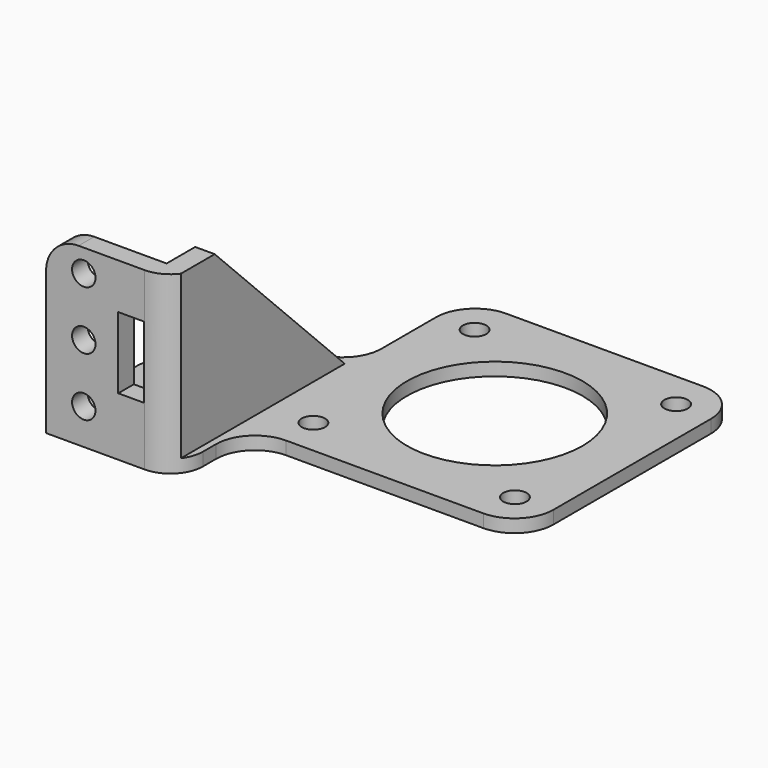
from build123d import *

# Parameters (mm, degrees)
F0_R         = 1.8
F0_R_2       = 13.5
F0_W         = 20.1372796029
F0_H         = 13.5
F1_DEPTH     = 2
F2_W         = 3
F2_H         = 33.5
F3_DEPTH     = 27
F4_W         = 16.1372796029
F4_H         = 3
F5_DEPTH     = 25
F6_R         = 1.8
F6_W         = 4
F6_H         = 11
F7_DEPTH     = 25
F8_SIZE      = 25
F9_SIZE      = 14
F10_R        = 5
F11_T1_DEPTH = 2
F11_T3_DEPTH = 32


# Not quite as in the source:
# - a fillet or chamfer that OpenCascade refuses, or shapes differently, is made with other operations: its cross-section is extruded or revolved along the edge and cut away or added


with BuildPart() as f1:
    # F0 (on Top) → F1 (new body)
    with BuildSketch(Plane.XY):
        Polygon((21.15, -21.15), (21.15, 21.15), (-21.15, 21.15), (-21.15, -1.15), (-21.15, -21.15), align=None)
        with Locations((-15.5, -15.5)):
            Circle(F0_R, mode=Mode.SUBTRACT)
        with Locations((15.5, -15.5)):
            Circle(F0_R, mode=Mode.SUBTRACT)
        with Locations((-15.5, 15.5)):
            Circle(F0_R, mode=Mode.SUBTRACT)
        Circle(F0_R_2, mode=Mode.SUBTRACT)
        with Locations((15.5, 15.5)):
            Circle(F0_R, mode=Mode.SUBTRACT)
        Polygon((-21.15, -21.15), (-21.15, -1.15), (-41.3, -1.15), (-41.3, -21.15), (-21.1627203971, -21.15), align=None)
        with Locations((-31.2313601986, -27.9)):
            Rectangle(F0_W, F0_H)
    extrude(amount=F1_DEPTH)

    # F2 (on Top) → F3 (join)
    with BuildSketch(Plane.XY):
        with Locations((-23.6627203971, -17.9)):
            Rectangle(F2_W, F2_H)
    extrude(amount=F3_DEPTH)

    # F4 (on face) → F5 (join)
    with BuildSketch(Plane.XY.offset(2)):
        with Locations((-33.2313601986, -33.15)):
            Rectangle(F4_W, F4_H)
    extrude(amount=F5_DEPTH)

    # F6 (on face) → F7 (cut)
    with BuildSketch(Plane(origin=(0, -31.65, 0), x_dir=(-1, 0, 0), z_dir=(0, 1, 0))):
        with Locations((35.5, 14.5)):
            Circle(F6_R)
        with Locations((35.5, 5.5)):
            Circle(F6_R)
        with Locations((35.5, 23.5)):
            Circle(F6_R)
        with Locations((28.2, 14.5)):
            Rectangle(F6_W, F6_H)
    extrude(amount=-F7_DEPTH, mode=Mode.SUBTRACT)

    # F8
    f8_edges = [f1.edges().sort_by_distance(p)[0] for p in [
        (-23.66272, -1.15, 27),
    ]]
    chamfer(f8_edges, length=F8_SIZE)

    # F9
    f9_edges = [f1.edges().sort_by_distance(p)[0] for p in [
        (-41.3, -1.15, 1),
    ]]
    chamfer(f9_edges, length=F9_SIZE)

    # F10
    f10_edges = [f1.edges().sort_by_distance(p)[0] for p in [
        (-41.3, -15.15, 1),
        (-27.3, -1.15, 1),
        (-21.16272, -34.65, 1),
        (-41.3, -33.15, 27),
    ]]
    fillet(f10_edges, radius=F10_R)

    # F11: fillet of radius 6 on 5 edges, made by hand

    # F11_s2 → F11_t1 (join)
    with BuildSketch(Plane.XY):
        with BuildLine():
            ThreePointArc((-26.1021448299, -1.2268404777), (-22.5517867046, 0.826546392), (-21.15, 4.6809509491))
            Line((-21.15, 4.6809509491), (-20.55, 4.6809509491))
            Line((-20.55, 4.6809509491), (-20.55, -1.15))
            Line((-20.55, -1.15), (-21.15, -1.75))
            ThreePointArc((-21.15, -1.75), (-25.2289321881, -1.75), (-25.9973593129, -1.8176196204))
            Line((-25.9973593129, -1.8176196204), (-26.1021448299, -1.2268404777))
        make_face()
        with BuildLine():
            ThreePointArc((-15.1627203971, -21.15), (-19.4053610842, -22.9073593129), (-21.1627203971, -27.15))
            Line((-21.1627203971, -27.15), (-21.1627203971, -21.15))
            Line((-21.1627203971, -21.15), (-15.1627203971, -21.15))
        make_face()
    extrude(amount=F11_T1_DEPTH)

    # F11_s4 → F11_t3 (cut)
    with BuildSketch(Plane.XY.offset(-15)):
        with BuildLine():
            ThreePointArc((21.15, -15.15), (19.3926406871, -19.3926406871), (15.15, -21.15))
            Line((15.15, -21.15), (21.15, -21.15))
            Line((21.15, -21.15), (21.15, -15.15))
        make_face()
        with BuildLine():
            ThreePointArc((15.15, 21.15), (19.3926406871, 19.3926406871), (21.15, 15.15))
            Line((21.15, 15.15), (21.15, 21.15))
            Line((21.15, 21.15), (15.15, 21.15))
        make_face()
        with BuildLine():
            ThreePointArc((-21.15, 15.15), (-19.3926406871, 19.3926406871), (-15.15, 21.15))
            Line((-15.15, 21.15), (-21.15, 21.15))
            Line((-21.15, 21.15), (-21.15, 15.15))
        make_face()
    extrude(amount=F11_T3_DEPTH, mode=Mode.SUBTRACT)


solid = f1.part
